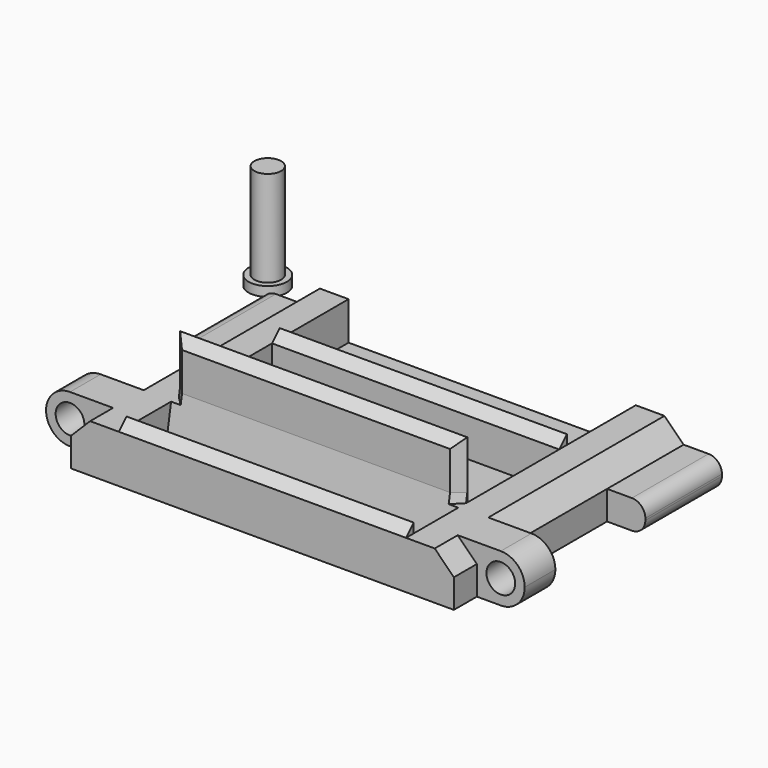
from build123d import *

# Parameters (mm, degrees)
F0_W         = 101.6
F0_H         = 76.2
F1_DEPTH     = 2.54
F2_W         = 12.7
F2_H         = 10.16
F3_DEPTH     = 12.7
F4_R         = 6.34999
F5_R         = 3.81
F6_DEPTH     = 25.4
F7_W         = 12.7
F7_H         = 76.2
F8_DEPTH     = 10.16
F9_SIZE      = 5.08
F10_W        = 76.2
F10_H        = 2.54
F11_DEPTH    = 12.7
F12_DEPTH    = 12.7
F14_DEPTH    = 2.54
F15_T4_DEPTH = 76.2
F16_SIZE     = 2.53999
F17_SIZE     = 2.53999
F18_R        = 5.08
F19_DEPTH    = 2.54
F20_R        = 3.556
F21_DEPTH    = 25.4
F22_W        = 10.16
F22_H        = 25.4
F23_DEPTH    = 7.62
F24_R        = 3.556


# Not quite as in the source:
# - a fillet or chamfer that OpenCascade refuses, or shapes differently, is made with other operations: its cross-section is extruded or revolved along the edge and cut away or added
# - a fillet or chamfer is up to 0.001 mm smaller than in the source, because OpenCascade refuses the exact size


with BuildPart() as f1:
    # F0 (on Top) → F1 (new body)
    with BuildSketch(Plane.XY):
        Rectangle(F0_W, F0_H)
    extrude(amount=F1_DEPTH)

    # F2 (on Top) → F3 (join)
    with BuildSketch(Plane.XY):
        with Locations((-57.15, -25.4)):
            Rectangle(F2_W, F2_H)
        with Locations((57.15, -25.4)):
            Rectangle(F2_W, F2_H)
    extrude(amount=F3_DEPTH)

    # F4 (radius 6.35 in the source; OpenCascade refuses exactly that, so slightly less here)
    f4_edges = [f1.edges().sort_by_distance(p)[0] for p in [
        (-63.5, -25.4, 12.7),
        (-63.5, -25.4, 0),
        (63.5, -25.4, 12.7),
        (63.5, -25.4, 0),
    ]]
    fillet(f4_edges, radius=F4_R)

    # F5 (on face) → F6 (cut)
    with BuildSketch(Plane.XZ.offset(30.48)):
        with Locations((-57.15, 6.35)):
            Circle(F5_R)
        with Locations((57.15, 6.35)):
            Circle(F5_R)
    extrude(amount=-F6_DEPTH, mode=Mode.SUBTRACT)

    # F7 (on face) → F8 (join)
    with BuildSketch(Plane.XY.offset(2.54)):
        with Locations((-44.45, 0)):
            Rectangle(F7_W, F7_H)
        with Locations((44.45, 0)):
            Rectangle(F7_W, F7_H)
    extrude(amount=F8_DEPTH)

    # F9
    f9_edges = [f1.edges().sort_by_distance(p)[0] for p in [
        (-50.8, 8.89, 12.7),
        (-50.8, -34.29, 12.7),
        (50.8, 8.89, 12.7),
        (50.8, -34.29, 12.7),
    ]]
    chamfer(f9_edges, length=F9_SIZE)

    # F10 (on face) → F11 (join)
    with BuildSketch(Plane.XY.offset(2.54)):
        with Locations((0, -36.83)):
            Rectangle(F10_W, F10_H)
        with Locations((0, 13.97)):
            Rectangle(F10_W, F10_H)
        with Locations((0, -19.05)):
            Rectangle(F10_W, F10_H)
    extrude(amount=F11_DEPTH)

    # F12 (add): a face of the model
    f12_faces = [f1.faces().sort_by_distance(p)[0] for p in [
        (0, -19.05, 15.24),
    ]]
    extrude(f12_faces, amount=F12_DEPTH)

    # F13 (on face) → F14 (join)
    with BuildSketch(Plane.XZ.offset(20.32)):
        Polygon((-38.1, 12.7), (-38.1, 2.54), (38.1, 2.54), (38.1, 12.7), (38.1, 15.24), (-38.1, 15.24), align=None)
    extrude(amount=F14_DEPTH)

    # F15: chamfer of 2.54 x 14.4050558218 on 1 edges, made by hand


with BuildPart() as f15_tool2:
    # F15_s3 → F15_t4 (new body)
    with BuildSketch(Plane.YZ.offset(38.1)):
        with BuildLine():
            Line((-22.9600564677, 0.2674957519), (-20.2199435323, 15.8074484262))
            Line((-20.2199435323, 15.8074484262), (-20.2199435323, 16.0955495427))
            ThreePointArc((-20.2199435323, 16.0955495427), (-21.5399717661, 15.5281011164), (-22.86, 15.5281011164))
            Line((-22.86, 15.5281011164), (-23.1481011164, 15.24))
            ThreePointArc((-23.1481011164, 15.24), (-23.1481011164, 7.753747876), (-23.2481575841, 0.2674957519))
            Line((-23.2481575841, 0.2674957519), (-22.9600564677, 0.2674957519))
        make_face()
    extrude(amount=-F15_T4_DEPTH)

    split(bisect_by=Plane.XY.offset(2.54), keep=Keep.TOP)

    split(bisect_by=Plane.XZ.offset(20.32), keep=Keep.TOP)


with BuildPart() as f1_1:
    add(f1.part)

    # F15_t1: cut F15_tool2
    add(f15_tool2.part, mode=Mode.SUBTRACT)

    # F16 (size 2.54 in the source; OpenCascade refuses exactly that, so slightly less here)
    f16_edges = [f1_1.edges().sort_by_distance(p)[0] for p in [
        (0, -20.32, 27.94),
        (0, -38.1, 15.24),
        (0, 12.7, 15.24),
    ]]
    chamfer(f16_edges, length=F16_SIZE)

    # F17 (size 2.54 in the source; OpenCascade refuses exactly that, so slightly less here)
    f17_edges = [f1_1.edges().sort_by_distance(p)[0] for p in [
        (-38.1, -20.32, 20.320005),
        (-38.1, -20.543935, 13.97),
        (38.1, -20.32, 20.320005),
        (38.1, -20.543935, 13.97),
    ]]
    chamfer(f17_edges, length=F17_SIZE)

    # F22 (on Top) → F23 (join)
    with BuildSketch(Plane.XY):
        Polygon((-50.8, 12.7), (-50.8, 38.1), (-60.96, 38.1), (-60.96, 12.5502143055), (-50.8, 12.5502143055), align=None)
        with Locations((55.88, 25.4)):
            Rectangle(F22_W, F22_H)
    extrude(amount=F23_DEPTH)

    # F24
    f24_edges = [f1_1.edges().sort_by_distance(p)[0] for p in [
        (-60.96, 25.325107, 7.62),
        (-60.96, 25.325107, 0),
        (60.96, 25.4, 7.62),
        (60.96, 25.4, 0),
    ]]
    fillet(f24_edges, radius=F24_R)


with BuildPart() as f19:
    # F18 (on Top) → F19 (new body)
    with BuildSketch(Plane.XY):
        with Locations((-70.2030956745, 51.4264591038)):
            Circle(F18_R)
    extrude(amount=F19_DEPTH)

    # F20 (on face) → F21 (join)
    with BuildSketch(Plane.XY.offset(2.54)):
        with Locations((-70.2030956745, 51.4264591038)):
            Circle(F20_R)
    extrude(amount=F21_DEPTH)


solid = Compound([f1_1.part, f19.part])
